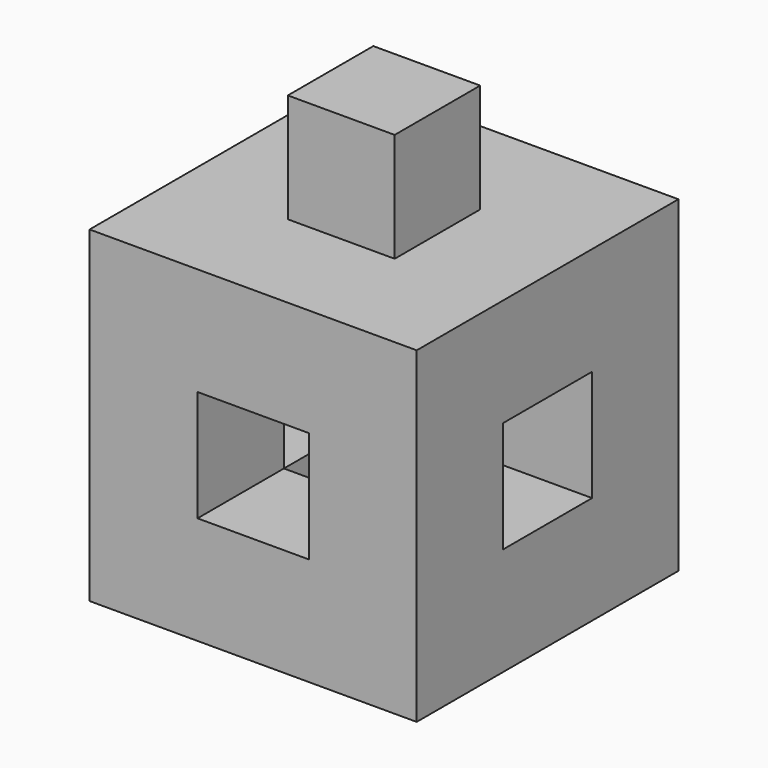
from build123d import *

# Parameters (mm, degrees)
F0_W         = 30
F0_H         = 30
F1_DEPTH     = 15
F2_W         = 9.8
F2_H         = 9.8
F3_DEPTH     = 10
F4_W         = 10.2
F4_H         = 10.2
F5_DEPTH     = 21
F6_W         = 10.2
F6_H         = 10.2
F7_DEPTH     = 30
F8_W         = 10.2
F8_H         = 10.2
F9_DEPTH     = 30.001
F10_T1_DEPTH = 20.9121426428
F10_T3_DEPTH = 20.9121426428


# Not quite as in the source:
# - a fillet or chamfer that OpenCascade refuses, or shapes differently, is made with other operations: its cross-section is extruded or revolved along the edge and cut away or added


with BuildPart() as f1:
    # F0 (on Front) → F1 (new body, symmetric)
    with BuildSketch(Plane.XZ):
        Rectangle(F0_W, F0_H)
    extrude(amount=F1_DEPTH, both=True)

    # F2 (on face) → F3 (join)
    with BuildSketch(Plane.XY.offset(15)):
        Rectangle(F2_W, F2_H)
    extrude(amount=F3_DEPTH)

    # F4 (on face) → F5 (cut)
    with BuildSketch(Plane(origin=(0, 0, -15), x_dir=(1, 0, 0), z_dir=(0, 0, -1))):
        Rectangle(F4_W, F4_H)
    extrude(amount=-F5_DEPTH, mode=Mode.SUBTRACT)

    # F6 (on face) → F7 (cut)
    with BuildSketch(Plane.YZ.offset(15)):
        Rectangle(F6_W, F6_H)
    extrude(amount=-F7_DEPTH, mode=Mode.SUBTRACT)

    # F8 (on face) → F9 (cut, through all)
    with BuildSketch(Plane.XZ.offset(15)):
        Rectangle(F8_W, F8_H)
    extrude(amount=-F9_DEPTH, mode=Mode.SUBTRACT)

    # F10: fillet of radius 3 on 4 edges, made by hand

    # F10_s2 → F10_t1 (join)
    with BuildSketch(Plane.YZ.offset(-10.4560713214)):
        with BuildLine():
            ThreePointArc((-5.1, 5.1), (-4.1194664753, 5.7658633372), (-2.9575714714, 6))
            Line((-2.9575714714, 6), (-5.1, 6))
            Line((-5.1, 6), (-5.1, 5.1))
        make_face()
        with BuildLine():
            ThreePointArc((5.1, 5.1), (4.1194664753, 5.7658633372), (2.9575714714, 6))
            Line((2.9575714714, 6), (5.1, 6))
            Line((5.1, 6), (5.1, 5.1))
        make_face()
    extrude(amount=F10_T1_DEPTH)

    # F10_s4 → F10_t3 (join)
    with BuildSketch(Plane.XZ.offset(-10.4560713214)):
        with BuildLine():
            ThreePointArc((5.1, 5.1), (4.1194664753, 5.7658633372), (2.9575714714, 6))
            Line((2.9575714714, 6), (5.1, 6))
            Line((5.1, 6), (5.1, 5.1))
        make_face()
        with BuildLine():
            ThreePointArc((-2.9575714714, 6), (-4.1194664753, 5.7658633372), (-5.1, 5.1))
            Line((-5.1, 5.1), (-5.1, 6))
            Line((-5.1, 6), (-2.9575714714, 6))
        make_face()
    extrude(amount=F10_T3_DEPTH)


solid = f1.part
